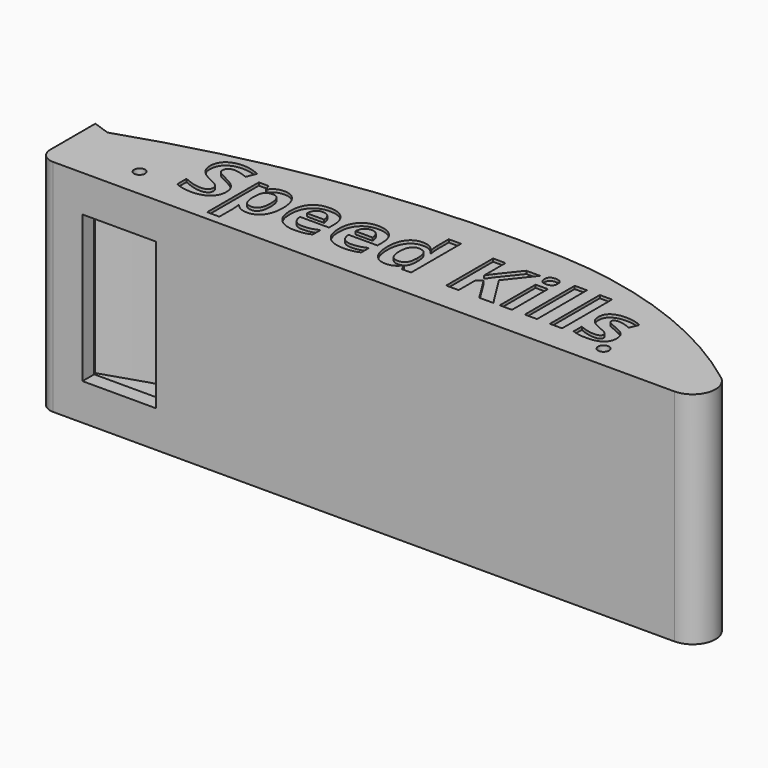
from build123d import *

# Parameters (mm, degrees)
F1_DEPTH     = 38.1
F3_DEPTH     = 38.1
F4_T         = -2.54
F5_W         = 12.7
F5_H         = 25.4
F6_DEPTH     = 6.35
F8_D         = 1.905
F9_TEXT_SIZE = 14.2131032875
F10_DEPTH    = 0.508


# Not quite as in the source:
# - Text() gives the source's letters only with a copy of the font that has no kerning and outlines rounded to 1/6400 em; it was checked with that copy


with BuildPart() as f1:
    # F0 (on Top) → F1 (new body)
    with BuildSketch(Plane.XY):
        with BuildLine():
            ThreePointArc((0, 2.54), (0.7439487758, 0.7439487758), (2.54, 0))
            Line((2.54, 0), (110.0765120345, 0))
            ThreePointArc((110.0765120345, 0), (113.8254855694, 2.6904351017), (112.4767437187, 7.1033863842))
            ThreePointArc((112.4767437187, 7.1033863842), (94.1856144859, 17.1277846685), (73.7459659576, 21.2840735912))
            ThreePointArc((73.7459659576, 21.2840735912), (36.3264056364, 19.4539531677), (0, 10.2907065302))
            Line((0, 10.2907065302), (0, 2.54))
        make_face()
    extrude(amount=F1_DEPTH)

    # F2 (on face) → F3 (join)
    with BuildSketch(Plane(origin=(0, 0, 0), x_dir=(1, 0, 0), z_dir=(0, 0, -1))):
        with BuildLine():
            ThreePointArc((2.9044583973, -11.3118282259), (1.4501533633, -10.8071718431), (0, -10.2907065302))
            Line((0, -10.2907065302), (0, -12.3227065302))
            Line((0, -12.3227065302), (2.9044583973, -11.3118282259))
        make_face()
    extrude(amount=-F3_DEPTH)

    # F4 (hollow: no face is removed)
    offset(amount=F4_T, kind=Kind.INTERSECTION, mode=Mode.SUBTRACT)

    # F5 (on face) → F6 (cut)
    with BuildSketch(Plane.XZ):
        with Locations((13.9760031201, 19.05)):
            Rectangle(F5_W, F5_H)
    extrude(amount=-F6_DEPTH, mode=Mode.SUBTRACT)

    # F8 (through all)
    with Locations(Plane.XY.offset(38.1)):
        with Locations((13.4439487758, 5.08), (94.7754855694, 3.81)):
            Hole(F8_D / 2)

    # F9 (on face) → F10 (cut)
    with BuildSketch(Plane.XY.offset(38.1)):
        with Locations((19.05, 4.9395287827)):
            Text('Speed Kills', F9_TEXT_SIZE, font='Open Sans', font_style=FontStyle.BOLD, text_align=(TextAlign.LEFT, TextAlign.BOTTOM))
    extrude(amount=-F10_DEPTH, mode=Mode.SUBTRACT)


solid = f1.part
